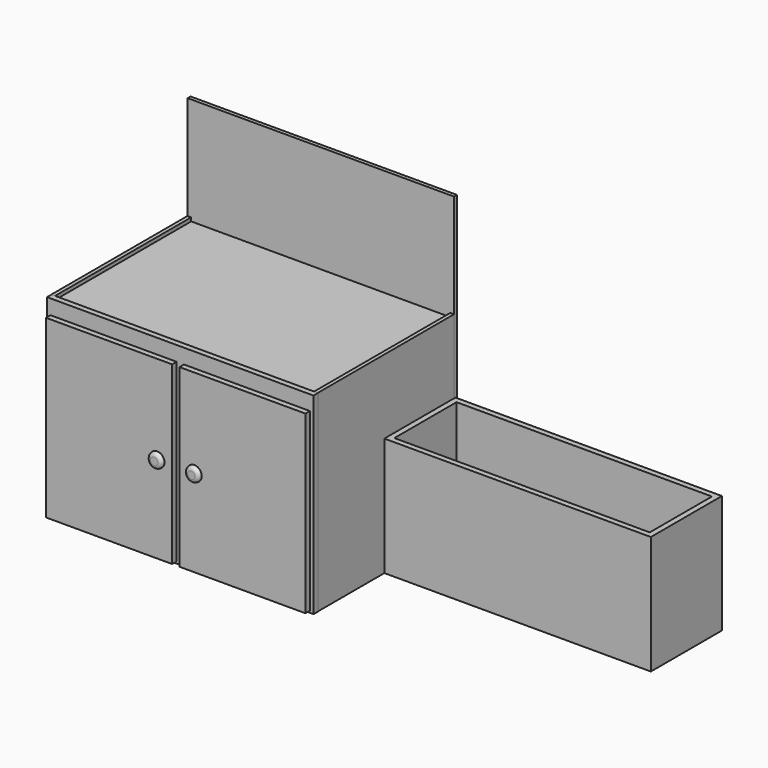
from build123d import *

# Parameters (mm, degrees)
F0_W      = 63.5
F0_H      = 457.2
F1_DEPTH  = 19.05
F2_W      = 584.2
F2_H      = 641.35
F2_H_2    = 19.05
F3_DEPTH  = 12.7
F4_W      = 583.9663306236
F4_H      = 19.05
F4_W_2    = 0.2336693764
F4_H_2    = 640.9677320718
F5_DEPTH  = 12.7
F6_W      = 914.4
F6_H      = 1016
F7_DEPTH  = 12.7
F8_W      = 25.4
F8_H      = 577.85
F8_W_2    = 406.4
F8_H_2    = 50.8
F9_DEPTH  = 19.05
F10_W     = 431.8
F10_H     = 603.25
F10_W_2   = 406.4
F10_H_2   = 577.85
F10_W_3   = 432.5660707131
F10_H_3   = 263.525
F11_DEPTH = 19.05
F12_R     = 25.4
F13_DEPTH = 12.7
F14_R     = 12.69999
F15_W     = 304.8
F15_H     = 406.4
F16_DEPTH = 914.4
F17_W     = 876.3
F17_H     = 266.7
F19_DEPTH = 387.35
F20_W     = 63.5
F20_H     = 457.2
F21_DEPTH = 19.05
F22_W     = 19.05
F22_H     = 63.5
F23_DEPTH = 596.9
F24_W     = 889
F24_H     = 584.2
F25_DEPTH = 12.7


# Not quite as in the source:
# - a fillet or chamfer is up to 0.001 mm smaller than in the source, because OpenCascade refuses the exact size
# - a feature names something its author has since deleted; it is built from what else it names


with BuildPart() as f1:
    # F0 (on Top) → F1 (new body)
    with BuildSketch(Plane.XY):
        Polygon((0, 63.5), (0, 0), (889, 0), (889, 63.5), (825.5, 63.5), (63.5, 63.5), align=None)
        with Locations((31.75, 292.1)):
            Rectangle(F0_W, F0_H)
        with Locations((857.25, 292.1)):
            Rectangle(F0_W, F0_H)
        Polygon((0, 584.2), (0, 520.7), (63.5, 520.7), (825.5, 520.7), (889, 520.7), (889, 584.2), align=None)
    extrude(amount=F1_DEPTH)

    # F22 (on face) → F23 (join, through all)
    with BuildSketch(Plane.XY.offset(19.05)):
        with Locations((431.8, 31.75)):
            Rectangle(F22_W, F22_H)
        with Locations((431.8, 552.45)):
            Rectangle(F22_W, F22_H)
    extrude(amount=F23_DEPTH)


with BuildPart() as f3:
    # F2 (on face) → F3 (new body)
    with BuildSketch(Plane.YZ.offset(889)):
        with Locations((292.1, 339.725)):
            Rectangle(F2_W, F2_H)
        with Locations((292.1, 9.525)):
            Rectangle(F2_W, F2_H_2)
    extrude(amount=F3_DEPTH)


with BuildPart() as f5:
    # F4 (on face) → F5 (new body)
    with BuildSketch(Plane(origin=(0, 0, 0), x_dir=(0, -1, 0), z_dir=(-1, 0, 0))):
        with Locations((-291.9831653118, 9.525)):
            Rectangle(F4_W, F4_H)
        with Locations((-584.0831653118, 9.525)):
            Rectangle(F4_W_2, F4_H)
        with Locations((-291.9831653118, 339.5338660359)):
            Rectangle(F4_W, F4_H_2)
    extrude(amount=F5_DEPTH)


with BuildPart() as f7:
    # F6 (on face) → F7 (new body)
    with BuildSketch(Plane(origin=(0, 584.2, 0), x_dir=(-1, 0, 0), z_dir=(0, 1, 0))):
        with Locations((-444.9155238152, 508)):
            Rectangle(F6_W, F6_H)
    extrude(amount=F7_DEPTH)


with BuildPart() as f9:
    # F8 (on face) → F9 (new body)
    with BuildSketch(Plane.XZ):
        Polygon((-11.9339292869, 19.05), (-11.9339292869, 0), (902.4660707131, 0), (902.4660707131, 19.05), (877.0660707131, 19.05), (470.6660707131, 19.05), (419.8660707131, 19.05), (13.4660707131, 19.05), align=None)
        Polygon((-11.9339292869, 596.9), (-11.9339292869, 19.05), (13.4660707131, 19.05), (13.4660707131, 282.575), (13.4660707131, 333.375), (13.4660707131, 596.9), align=None)
        with Locations((889.7660707131, 307.975)):
            Rectangle(F8_W, F8_H)
        Polygon((-11.9339292869, 660.4), (-11.9339292869, 596.9), (13.4660707131, 596.9), (419.8660707131, 596.9), (470.6660707131, 596.9), (877.0660707131, 596.9), (902.4660707131, 596.9), (902.4660707131, 660.4), align=None)
        Polygon((419.8660707131, 282.575), (419.8660707131, 19.05), (470.6660707131, 19.05), (470.6660707131, 596.9), (419.8660707131, 596.9), (419.8660707131, 333.375), align=None)
        with Locations((216.6660707131, 307.975)):
            Rectangle(F8_W_2, F8_H_2)
    extrude(amount=F9_DEPTH)

    # F10 (on face) → F11 (join)
    with BuildSketch(Plane.XZ.offset(19.05)):
        with Locations((673.8660707131, 307.975)):
            Rectangle(F10_W, F10_H)
        with Locations((673.8660707131, 307.975)):
            Rectangle(F10_W_2, F10_H_2, mode=Mode.SUBTRACT)
        with Locations((673.8660707131, 307.975)):
            Rectangle(F10_W_2, F10_H_2)
        with Locations((216.2830353566, 307.975)):
            Rectangle(F10_W_3, F10_H)
        with Locations((216.6660707131, 150.8125)):
            Rectangle(F10_W_2, F10_H_3, mode=Mode.SUBTRACT)
        with Locations((216.6660707131, 465.1375)):
            Rectangle(F10_W_2, F10_H_3, mode=Mode.SUBTRACT)
        with Locations((216.6660707131, 465.1375)):
            Rectangle(F10_W_2, F10_H_3)
        with Locations((216.6660707131, 150.8125)):
            Rectangle(F10_W_2, F10_H_3)
    extrude(amount=F11_DEPTH)

    # F12 (on face) → F13 (join)
    with BuildSketch(Plane.XZ.offset(38.1)):
        with Locations((508.7660707131, 304.8)):
            Circle(F12_R)
        with Locations((381, 304.8)):
            Circle(F12_R)
    extrude(amount=F13_DEPTH)

    # F14 (radius 12.7 in the source; OpenCascade refuses exactly that, so slightly less here)
    f14_edges = [f9.edges().sort_by_distance(p)[0] for p in [
        (483.366071, -50.8, 304.8),
        (355.6, -50.8, 304.8),
    ]]
    fillet(f14_edges, radius=F14_R)


with BuildPart() as f16:
    # F15 (on face) → F16 (new body)
    with BuildSketch(Plane.YZ.offset(901.7)):
        with Locations((438.0083848, 203.2)):
            Rectangle(F15_W, F15_H)
    extrude(amount=F16_DEPTH)

    # F17 (on face) → F19 (cut, through all)
    with BuildSketch(Plane.XY.offset(406.4)):
        with Locations((1358.9, 438.0083848)):
            Rectangle(F17_W, F17_H)
    extrude(amount=-F19_DEPTH, mode=Mode.SUBTRACT)


with BuildPart() as f21:
    # F20 (on offset) → F21 (new body)
    with BuildSketch(Plane.XY.offset(635)):
        Polygon((0, 63.5), (0, 0), (889, 0), (889, 63.5), (825.5, 63.5), (63.5, 63.5), align=None)
        with Locations((31.75, 292.1)):
            Rectangle(F20_W, F20_H)
        with Locations((857.25, 292.1)):
            Rectangle(F20_W, F20_H)
        Polygon((0, 584.2), (0, 520.7), (63.5, 520.7), (825.5, 520.7), (889, 520.7), (889, 584.2), align=None)
    extrude(amount=-F21_DEPTH)


with BuildPart() as f25:
    # F24 (on face) → F25 (new body)
    with BuildSketch(Plane.XY.offset(635)):
        with Locations((444.5, 292.1)):
            Rectangle(F24_W, F24_H)
    extrude(amount=F25_DEPTH)


solid = Compound([f1.part, f3.part, f5.part, f7.part, f9.part, f16.part, f21.part, f25.part])
